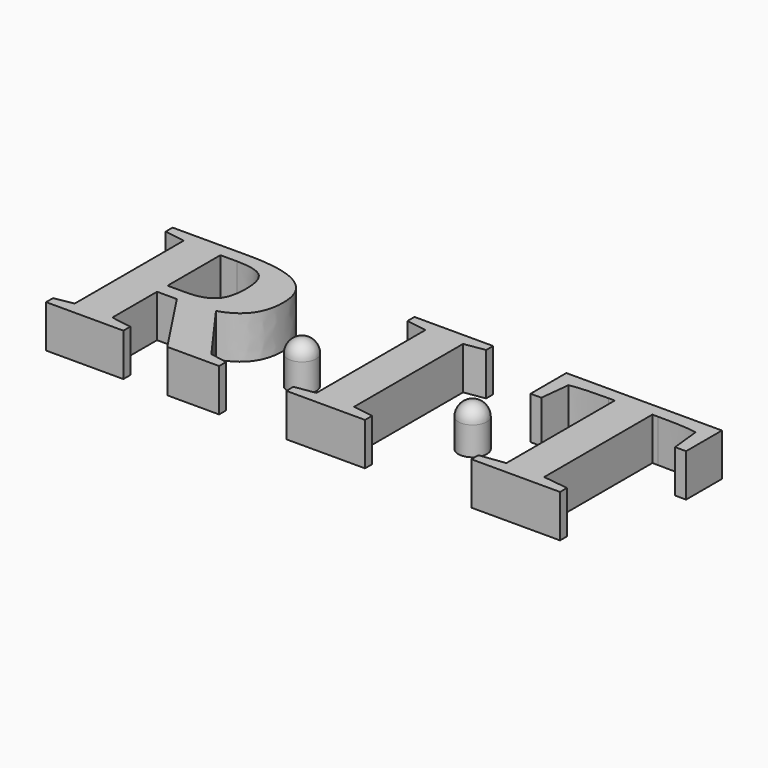
from build123d import *

# Parameters (mm, degrees)
F0_R         = 2.54
F0_TEXT_SIZE = 43.6842458851
F1_DEPTH     = 7.62
F2_R         = 2.54


# Not quite as in the source:
# - Text() gives the source's letters only with a copy of the font that has no kerning and outlines rounded to 1/6400 em; it was checked with that copy


with BuildPart() as f1:
    # F0 (on Top) → F1 (new body)
    with BuildSketch(Plane.XY):
        with Locations((35.56, -17.4826570373)):
            Circle(F0_R)
        with Locations((66.04, -17.4826570373)):
            Circle(F0_R)
        with Locations((0, -31.4526570373)):
            Text('R I T', F0_TEXT_SIZE, font='Tinos', font_style=FontStyle.BOLD, text_align=(TextAlign.LEFT, TextAlign.BOTTOM))
    extrude(amount=F1_DEPTH)

    # F2
    f2_edges = [f1.edges().sort_by_distance(p)[0] for p in [
        (33.02, -17.482657, 7.62),
        (63.5, -17.482657, 7.62),
    ]]
    fillet(f2_edges, radius=F2_R)


solid = f1.part
